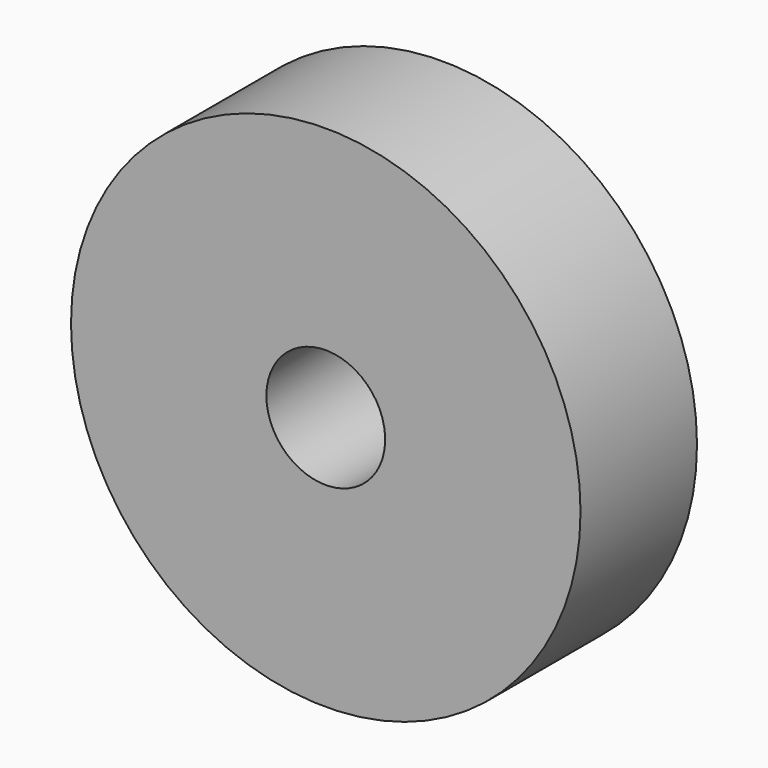
from build123d import *

# Parameters (mm, degrees)
F0_R     = 11.1125
F1_DEPTH = 6.35
F3_D     = 5.1816


# Not quite as in the source:
# - a length typed as a fraction of an inch, garbled in the dataset ("3 / 203.2 mm" for 3/8 in), is restored


with BuildPart() as f1:
    # F0 (on Front) → F1 (new body)
    with BuildSketch(Plane.XZ):
        Circle(F0_R)
    extrude(amount=F1_DEPTH)

    # F3 (through all)
    with Locations(Plane.XZ.offset(6.35)):
        with Locations((0, 0)):
            Hole(F3_D / 2)


solid = f1.part
